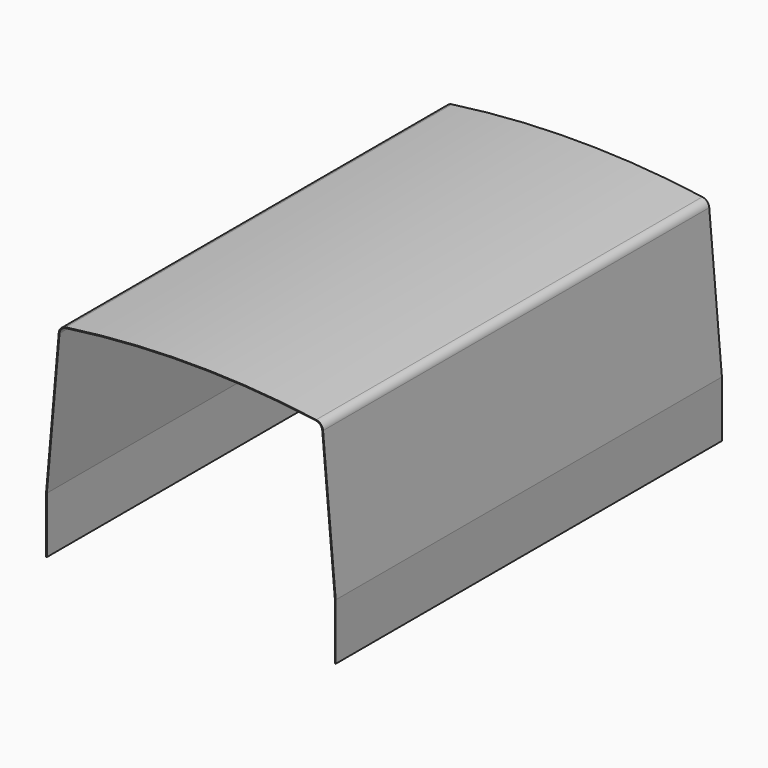
from build123d import *

# Parameters (mm, degrees)
F1_DEPTH = 3000
F3_DEPTH = 5
F4_DEPTH = 350


# Not quite as in the source:
# - ends of sketch curves that miss each other by under 0.0002 mm in the source are joined


with BuildPart() as f1:
    # F0 (on Front) → F1 (new body)
    with BuildSketch(Plane.XZ):
        with BuildLine():
            Line((-821.2220771658, 900.4357782981), (-900, 0))
            Line((-900, 0), (-894.9809055989, 0))
            Line((-894.9809055989, 0), (-816.2411084255, 900))
            ThreePointArc((-816.2411084255, 900), (-804.0533773431, 927.0548092338), (-777.6727873626, 940.6403884962))
            ThreePointArc((-777.6727873626, 940.6403884962), (0, 995.0000047684), (777.6727873915, 940.640388702))
            ThreePointArc((777.6727873915, 940.640388702), (804.0533773431, 927.0548092338), (816.2411084255, 900))
            Line((816.2411084255, 900), (894.9809008123, 0))
            Line((894.9809008123, 0), (900, 0))
            Line((900, 0), (821.2220771658, 900.4357782981))
            ThreePointArc((821.2220771658, 900.4357782981), (807.6801551758, 930.4966742615), (778.3683916368, 945.5917607313))
            ThreePointArc((778.3683916368, 945.5917607313), (0, 999.9999997922), (-778.3683916368, 945.5917607313))
            ThreePointArc((-778.3683916368, 945.5917607313), (-807.6801551758, 930.4966742615), (-821.2220771658, 900.4357782981))
        make_face()
    extrude(amount=F1_DEPTH)

    # F2 (on face) → F3 (join)
    with BuildSketch(Plane(origin=(0, 0, 0), x_dir=(-1, 0, 0), z_dir=(0, 1, 0))):
        with BuildLine():
            Line((-816.2411084255, 900), (-894.9809008123, 0))
            Line((-894.9809008123, 0), (894.9809055989, 0))
            Line((894.9809055989, 0), (816.2411084255, 900))
            ThreePointArc((816.2411084255, 900), (804.0533773431, 927.0548092338), (777.6727873626, 940.6403884962))
            ThreePointArc((777.6727873626, 940.6403884962), (-7.3e-09, 995.0000047684), (-777.6727873915, 940.640388702))
            ThreePointArc((-777.6727873915, 940.640388702), (-804.0533773182, 927.0548092601), (-816.2411084255, 900))
        make_face()
    extrude(amount=-F3_DEPTH)

    # F4 (add): a face of the model
    f4_faces = [f1.faces().sort_by_distance(p)[0] for p in [
        (898.4794719492, -1502.5, 0),
    ]]
    extrude(f4_faces, amount=F4_DEPTH)


solid = f1.part
